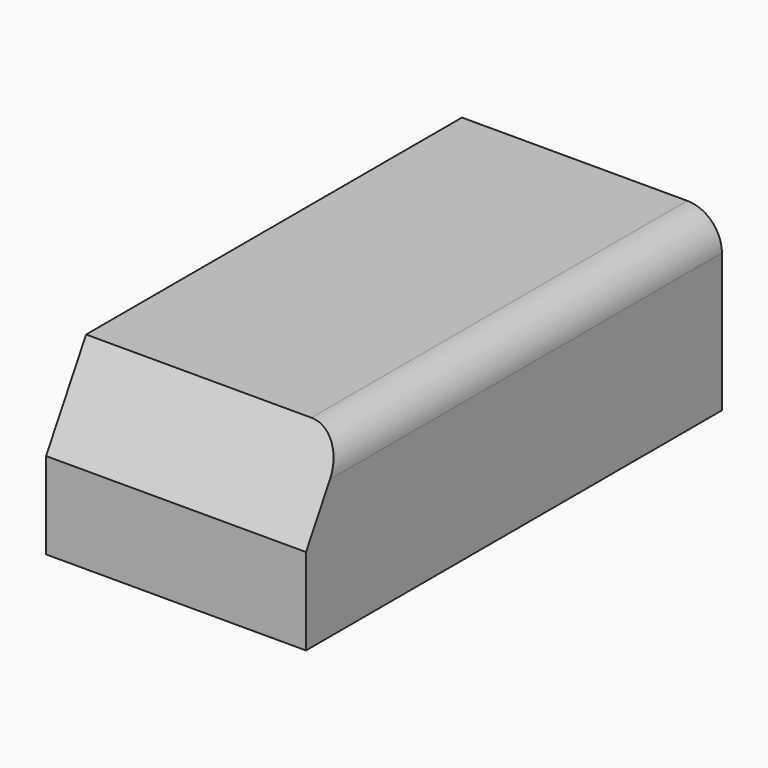
from build123d import *

# Parameters (mm, degrees)
F0_W        = 38.1
F0_H        = 76.2
F1_DEPTH    = 25.4
F2_R        = 5.08
F3_T1_DEPTH = 98.731978168
F3_T6_ANGLE = 90


# Not quite as in the source:
# - a fillet or chamfer that OpenCascade refuses, or shapes differently, is made with other operations: its cross-section is extruded or revolved along the edge and cut away or added


with BuildPart() as f1:
    # F0 (on Top) → F1 (new body)
    with BuildSketch(Plane.XY):
        Rectangle(F0_W, F0_H)
    extrude(amount=F1_DEPTH)

    # F2
    f2_edges = [f1.edges().sort_by_distance(p)[0] for p in [
        (19.05, 0, 25.4),
    ]]
    fillet(f2_edges, radius=F2_R)

    # F3: chamfer of 12.7 x 7.3323484187 on 1 edges, made by hand

    # F3_s2 → F3_t1 (cut)
    with BuildSketch(Plane.YZ.offset(-51.905989084)):
        Polygon((-38.1, 12.7), (-30.7676515813, 25.4), (-38.1, 25.4), align=None)
    extrude(amount=F3_T1_DEPTH, mode=Mode.SUBTRACT)


with BuildPart() as f3_tool4:
    # F3_s5 → F3_t6 (revolve)
    with BuildSketch(Plane.XY.offset(20.32)):
        Polygon((13.97, -33.7005909488), (19.05, -30.7676515813), (19.05, -38.1), (13.97, -38.1), align=None)
    revolve(axis=Axis((13.97, -38.1, 20.32), (0, -1, 0)), revolution_arc=F3_T6_ANGLE)

    split(bisect_by=Plane(origin=(0, -34.074261314, 19.6727839421), x_dir=(1, 0, 0), z_dir=(0, -0.8660254038, 0.5)), keep=Keep.TOP)


with BuildPart() as f1_1:
    add(f1.part)

    # F3_t3: cut F3_tool4
    add(f3_tool4.part, mode=Mode.SUBTRACT)


solid = f1_1.part
